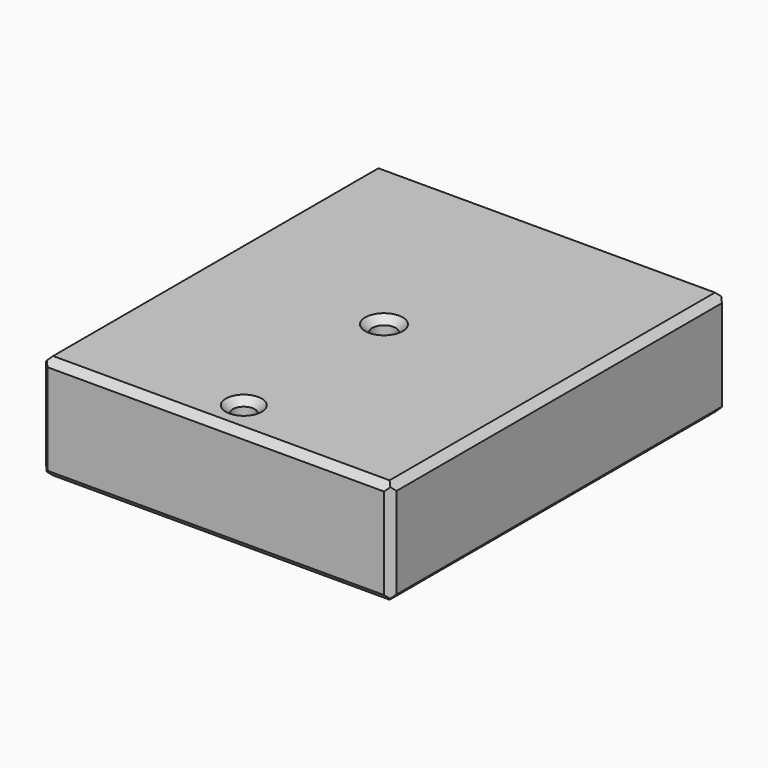
from build123d import *

# Parameters (mm, degrees)
F0_W        = 127
F0_H        = 152.4
F0_R        = 4.25
F1_DEPTH    = 38.1
F3_R        = 3.96875
F4_DEPTH    = 50.8
F5_R        = 6.25
F5_R_2      = 4.25
F5_R_3      = 5.96875
F5_R_4      = 3.96875
F6_DEPTH    = 12.7
F7_C1_SIZE  = 2.54
F7_C2_SIZE  = 2.54
F7_C3_SIZE  = 2.54
F7_C4_SIZE  = 2.54
F7_C5_SIZE  = 2.54
F7_C6_SIZE  = 2.54
F7_C7_SIZE  = 2.54
F7_C8_SIZE  = 2.54
F7_C9_SIZE  = 2.54
F7_C10_SIZE = 2.54
F7_C11_SIZE = 2.54
F7_C12_SIZE = 2.54
F7_C13_SIZE = 2.54
F7_C14_SIZE = 2.54
F7_C15_SIZE = 2.54
F7_C16_SIZE = 2.54


# Not quite as in the source:
# - two fillets or chamfers of one size are made in one step
# - a feature names something its author has since deleted; it is built from what else it names


with BuildPart() as f1:
    # F0 (on Top) → F1 (new body)
    with BuildSketch(Plane.XY):
        Rectangle(F0_W, F0_H)
        Circle(F0_R, mode=Mode.SUBTRACT)
    extrude(amount=F1_DEPTH)

    # F3 (on face) → F4 (cut)
    with BuildSketch(Plane.XY.offset(38.1)):
        with Locations((0, -63.5)):
            Circle(F3_R)
    extrude(amount=-F4_DEPTH, mode=Mode.SUBTRACT)

    # F5 (on face) → F6 (cut)
    with BuildSketch(Plane(origin=(0, 0, 0), x_dir=(1, 0, 0), z_dir=(0, 0, -1))):
        Circle(F5_R)
        Circle(F5_R_2, mode=Mode.SUBTRACT)
        with Locations((0, 63.5)):
            Circle(F5_R_3)
        with Locations((0, 63.5)):
            Circle(F5_R_4, mode=Mode.SUBTRACT)
    extrude(amount=-F6_DEPTH, mode=Mode.SUBTRACT)

    # F7: chamfer of 2.54 on 16 edges, made by hand

    # F7_c1
    f7_c1_edges = [f1.edges().sort_by_distance(p)[0] for p in [
        (-63.5, -76.2, 19.05),
    ]]
    chamfer(f7_c1_edges, length=F7_C1_SIZE)

    # F7_c2
    f7_c2_edges = [f1.edges().sort_by_distance(p)[0] for p in [
        (63.5, -76.2, 19.05),
    ]]
    chamfer(f7_c2_edges, length=F7_C2_SIZE)

    # F7_c3
    f7_c3_edges = [f1.edges().sort_by_distance(p)[0] for p in [
        (0, -76.2, 0),
    ]]
    chamfer(f7_c3_edges, length=F7_C3_SIZE)

    # F7_c4
    f7_c4_edges = [f1.edges().sort_by_distance(p)[0] for p in [
        (0, -76.2, 38.1),
    ]]
    chamfer(f7_c4_edges, length=F7_C4_SIZE)

    # F7_c5
    f7_c5_edges = [f1.edges().sort_by_distance(p)[0] for p in [
        (-63.5, 76.2, 19.05),
    ]]
    chamfer(f7_c5_edges, length=F7_C5_SIZE)

    # F7_c6
    f7_c6_edges = [f1.edges().sort_by_distance(p)[0] for p in [
        (-63.5, 0, 0),
    ]]
    chamfer(f7_c6_edges, length=F7_C6_SIZE)

    # F7_c7
    f7_c7_edges = [f1.edges().sort_by_distance(p)[0] for p in [
        (-63.5, 0, 38.1),
    ]]
    chamfer(f7_c7_edges, length=F7_C7_SIZE)

    # F7_c8
    f7_c8_edges = [f1.edges().sort_by_distance(p)[0] for p in [
        (63.5, 76.2, 19.05),
    ]]
    chamfer(f7_c8_edges, length=F7_C8_SIZE)

    # F7_c9
    f7_c9_edges = [f1.edges().sort_by_distance(p)[0] for p in [
        (63.5, 0, 0),
    ]]
    chamfer(f7_c9_edges, length=F7_C9_SIZE)

    # F7_c10
    f7_c10_edges = [f1.edges().sort_by_distance(p)[0] for p in [
        (63.5, 0, 38.1),
    ]]
    chamfer(f7_c10_edges, length=F7_C10_SIZE)

    # F7_c11
    f7_c11_edges = [f1.edges().sort_by_distance(p)[0] for p in [
        (0, 76.2, 0),
    ]]
    chamfer(f7_c11_edges, length=F7_C11_SIZE)

    # F7_c12
    f7_c12_edges = [f1.edges().sort_by_distance(p)[0] for p in [
        (-5.96875, -63.5, 0),
    ]]
    chamfer(f7_c12_edges, length=F7_C12_SIZE)

    # F7_c13
    f7_c13_edges = [f1.edges().sort_by_distance(p)[0] for p in [
        (-6.25, 0, 0),
    ]]
    chamfer(f7_c13_edges, length=F7_C13_SIZE)

    # F7_c14
    f7_c14_edges = [f1.edges().sort_by_distance(p)[0] for p in [
        (0, 76.2, 38.1),
    ]]
    chamfer(f7_c14_edges, length=F7_C14_SIZE)

    # F7_c15
    f7_c15_edges = [f1.edges().sort_by_distance(p)[0] for p in [
        (-3.96875, -63.5, 38.1),
    ]]
    chamfer(f7_c15_edges, length=F7_C15_SIZE)

    # F7_c16
    f7_c16_edges = [f1.edges().sort_by_distance(p)[0] for p in [
        (-4.25, 0, 38.1),
    ]]
    chamfer(f7_c16_edges, length=F7_C16_SIZE)


solid = f1.part
